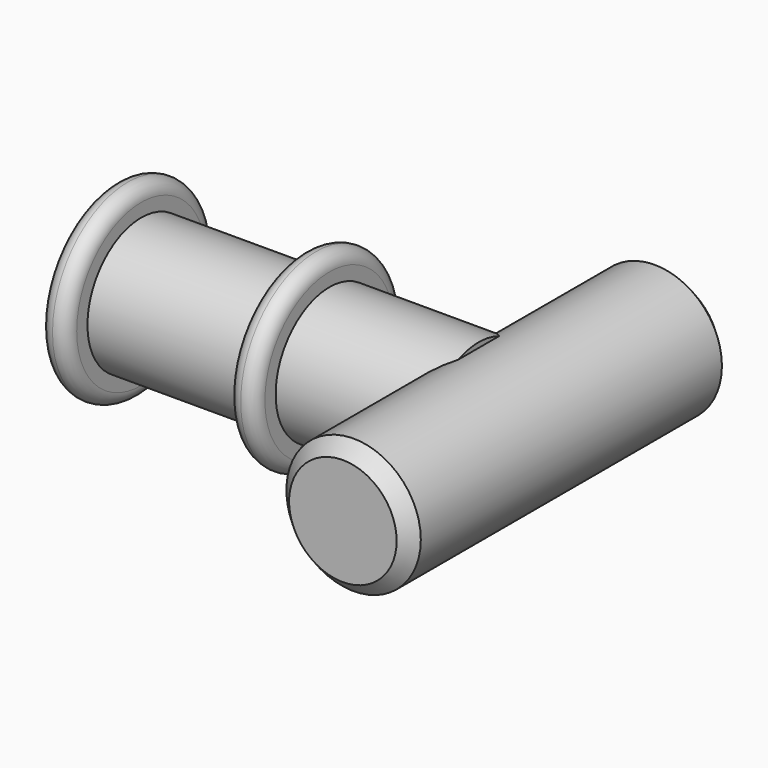
from build123d import *

# Parameters (mm, degrees)
F0_R      = 6.35
F1_DEPTH  = 15.24
F2_R      = 8.89
F3_DEPTH  = 2.54
F4_R      = 1.26999
F5_R      = 8.89
F6_DEPTH  = 2.54
F7_R      = 1.26999
F8_R      = 6.35
F9_DEPTH  = 19.05
F10_R     = 6.35
F11_DEPTH = 14.097
F12_SIZE  = 1.27


# Not quite as in the source:
# - a fillet or chamfer is up to 0.001 mm smaller than in the source, because OpenCascade refuses the exact size


with BuildPart() as f1:
    # F0 (on Right) → F1 (new body)
    with BuildSketch(Plane.YZ):
        with Locations((0, 182.4067449291)):
            Circle(F0_R)
    extrude(amount=F1_DEPTH)

    # F2 (on face) → F3 (join)
    with BuildSketch(Plane(origin=(0, 0, 0), x_dir=(0, -1, 0), z_dir=(-1, 0, 0))):
        with Locations((0, 182.4067449291)):
            Circle(F2_R)
    extrude(amount=F3_DEPTH)

    # F4 (radius 1.27 in the source; OpenCascade refuses exactly that, so slightly less here)
    f4_edges = [f1.edges().sort_by_distance(p)[0] for p in [
        (-1.27, -8.89, 182.406745),
        (0, 8.89, 182.406745),
        (-2.54, 8.89, 182.406745),
    ]]
    fillet(f4_edges, radius=F4_R)

    # F5 (on face) → F6 (join)
    with BuildSketch(Plane.YZ.offset(15.24)):
        with Locations((0, 182.4067449291)):
            Circle(F5_R)
    extrude(amount=F6_DEPTH)

    # F7 (radius 1.27 in the source; OpenCascade refuses exactly that, so slightly less here)
    f7_edges = [f1.edges().sort_by_distance(p)[0] for p in [
        (16.51, 8.89, 182.406745),
        (15.24, -8.89, 182.406745),
        (17.78, -8.89, 182.406745),
    ]]
    fillet(f7_edges, radius=F7_R)



with BuildPart() as f9:
    # F8 (on Front) → F9 (new body, symmetric)
    with BuildSketch(Plane.XZ):
        with Locations((34.29, 182.4067449291)):
            Circle(F8_R)
    extrude(amount=F9_DEPTH, both=True)


with BuildPart() as f1_1:
    add(f1.part)

    add(f9.part)  # F11 merges F9
    # F10 (on face) → F11 (join)
    with BuildSketch(Plane.YZ.offset(17.78)):
        with Locations((0, 182.4067449291)):
            Circle(F10_R)
    extrude(amount=F11_DEPTH)

    # F12
    f12_edges = [f1_1.edges().sort_by_distance(p)[0] for p in [
        (27.94, -19.05, 182.406745),
        (27.94, 19.05, 182.406745),
    ]]
    chamfer(f12_edges, length=F12_SIZE)


with BuildPart() as f1_2:
    # F14: moved
    add(f1_1.part.moved(Location((-15.24, 0, -182.4067449291))))


solid = f1_2.part
